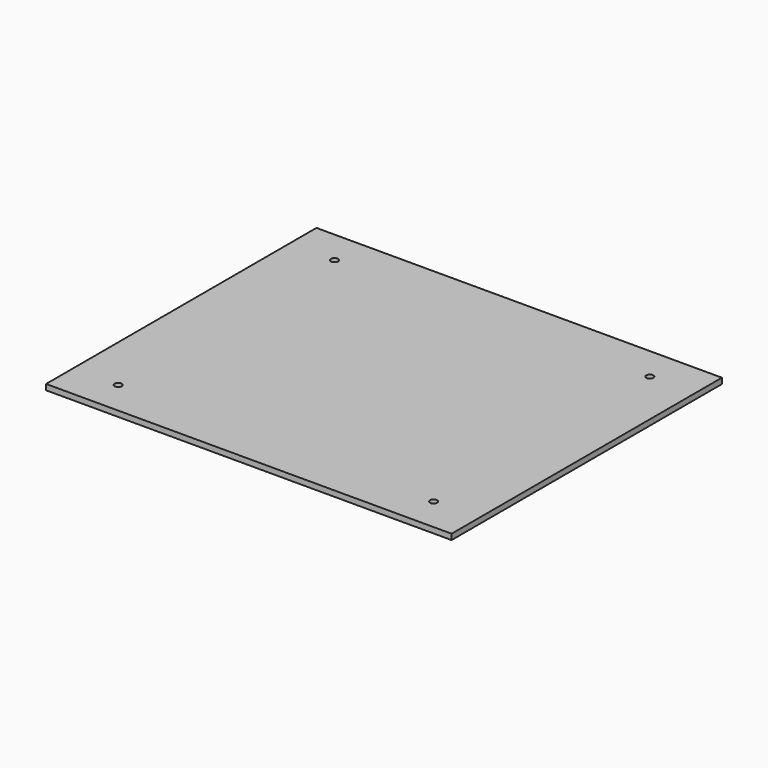
from build123d import *

# Parameters (mm, degrees)
F0_W     = 228.6
F0_H     = 190.5
F0_R     = 2
F1_DEPTH = 3.175


# Not quite as in the source:
# - a length typed as a fraction of an inch, garbled in the dataset ("3 / 203.2 mm" for 3/8 in), is restored


with BuildPart() as f1:
    # F0 (on Top) → F1 (new body)
    with BuildSketch(Plane.XY):
        with Locations((-493.4600528501, -289.4775138378)):
            Rectangle(F0_W, F0_H)
        with Locations((-582.3600528501, -365.6775138378)):
            Circle(F0_R, mode=Mode.SUBTRACT)
        with Locations((-404.5600528501, -365.6775138378)):
            Circle(F0_R, mode=Mode.SUBTRACT)
        with Locations((-582.3600528501, -213.2775138378)):
            Circle(F0_R, mode=Mode.SUBTRACT)
        with Locations((-404.5600528501, -213.2775138378)):
            Circle(F0_R, mode=Mode.SUBTRACT)
    extrude(amount=F1_DEPTH)


solid = f1.part
